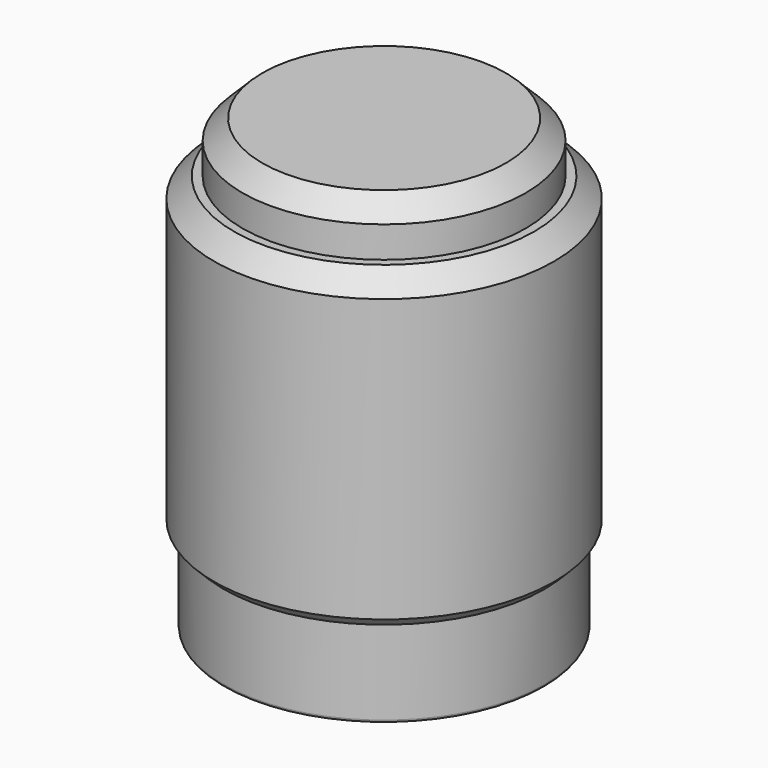
from build123d import *

# Parameters (mm, degrees)
F2_S7_R     = 5.66
F2_T8_DEPTH = 10
F3_R        = 0.1
F4_D        = 2.2606
F4_DEPTH    = 6.001


# Not quite as in the source:
# - a fillet or chamfer that OpenCascade refuses, or shapes differently, is made with other operations: its cross-section is extruded or revolved along the edge and cut away or added


with BuildPart() as f1:
    # F0 (on Front) → F1 (revolve)
    with BuildSketch(Plane.XZ):
        Polygon((4.75, 4), (4.75, 0), (5.66, 0), (5.66, 2.7), (6, 2.7), (6, 14.05), (5, 14.05), (5, 15.85), (0, 15.85), (0, 12.954), (1.61, 12.954), (1.61, 4), align=None)
    revolve(axis=Axis((0, 0, 9.925), (0, 0, 1)))

    # F2: chamfer of 0.7 on 3 edges, made by hand

    # F2_s1 → F2_t2 (revolve, cut)
    with BuildSketch(Plane.XZ):
        Polygon((6, 13.35), (5.3, 14.05), (6, 14.05), align=None)
    revolve(axis=Axis((0, 0, 14.05), (0, 0, 1)), mode=Mode.SUBTRACT)


with BuildPart() as f2_tool4:
    # F2_s5 → F2_t6 (revolve)
    with BuildSketch(Plane.XZ):
        Polygon((5.3, 2.7), (6, 3.4), (6, 2.7), align=None)
    revolve(axis=Axis((0, 0, 2.7), (0, 0, 1)))

    # F2_s7 → F2_t8 (cut, symmetric)
    with BuildSketch(Plane.XY.offset(3.1)):
        Circle(F2_S7_R)
    extrude(amount=F2_T8_DEPTH, both=True, mode=Mode.SUBTRACT)


with BuildPart() as f1_1:
    add(f1.part)

    # F2_t3: cut F2_tool4
    add(f2_tool4.part, mode=Mode.SUBTRACT)

    # F2_s9 → F2_t10 (revolve, cut)
    with BuildSketch(Plane.XZ):
        Polygon((5, 15.15), (4.3, 15.85), (5, 15.85), align=None)
    revolve(axis=Axis((0, 0, 15.85), (0, 0, 1)), mode=Mode.SUBTRACT)

    # F3
    f3_edges = [f1_1.edges().sort_by_distance(p)[0] for p in [
        (-5.66, 0, 0),
    ]]
    fillet(f3_edges, radius=F3_R)

    # F4 (through all, one way)
    with BuildSketch(Plane.XZ):
        with Locations((0, 7.239)):
            Circle(F4_D / 2)
    extrude(amount=-F4_DEPTH, mode=Mode.SUBTRACT)


solid = f1_1.part
